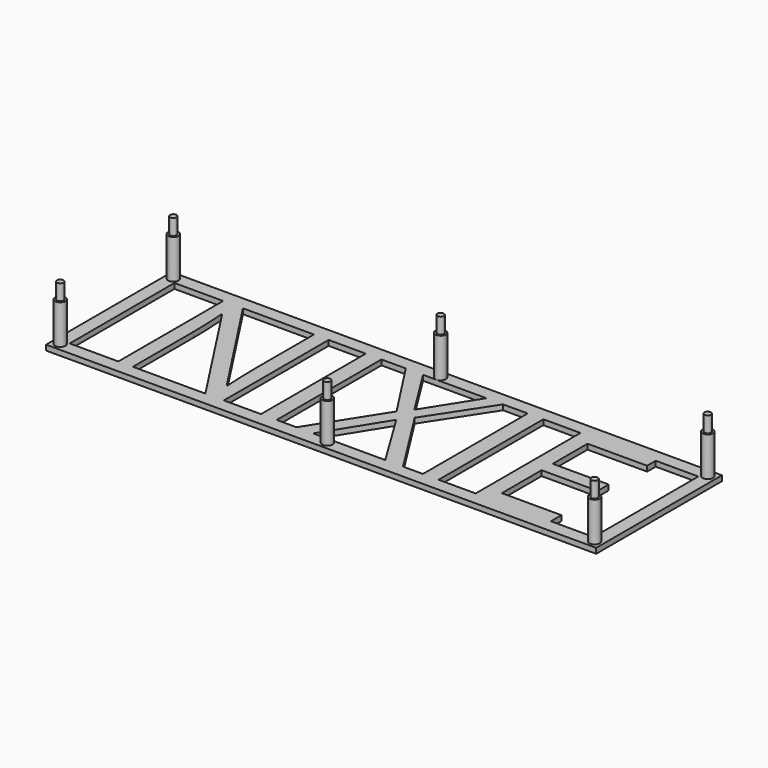
from build123d import *

# Parameters (mm, degrees)
F0_W          = 210
F0_H          = 60
F0_W_2        = 200
F0_H_2        = 50
F1_DEPTH      = 2
F2_R          = 2
F3_DEPTH      = 15
F4_R          = 1.25
F5_DEPTH      = 6
F6_R          = 1.25
F7_DEPTH      = 6
F8_R          = 1.25
F9_DEPTH      = 6
F10_R         = 1.25
F11_DEPTH     = 6
F12_TEXT_SIZE = 72.2222222222
F13_DEPTH     = 2
F14_R         = 1.25
F15_DEPTH     = 6
F16_R         = 1.25
F17_DEPTH     = 6


# Not quite as in the source:
# - a feature names something its author has since deleted; it is built from what else it names
# - Text() gives the source's letters only with a copy of the font that has no kerning and outlines rounded to 1/6400 em; it was checked with that copy


with BuildPart() as f1:
    # F0 (on Top) → F1 (new body)
    with BuildSketch(Plane.XY):
        with Locations((-105, 30)):
            Rectangle(F0_W, F0_H)
        with Locations((-105, 30)):
            Rectangle(F0_W_2, F0_H_2, mode=Mode.SUBTRACT)
    extrude(amount=F1_DEPTH)

    # F2 (on face) → F3 (join)
    with BuildSketch(Plane.XY.offset(2)):
        with Locations((-207, 3)):
            Circle(F2_R)
        with Locations((-207, 57)):
            Circle(F2_R)
        with Locations((-3, 57)):
            Circle(F2_R)
        with Locations((-3, 3)):
            Circle(F2_R)
        with Locations((-105, 3)):
            Circle(F2_R)
        with Locations((-105, 57)):
            Circle(F2_R)
    extrude(amount=F3_DEPTH)

    # F4 (on face) → F5 (join)
    with BuildSketch(Plane.XY.offset(17)):
        with Locations((-207, 3)):
            Circle(F4_R)
    extrude(amount=F5_DEPTH)

    # F6 (on face) → F7 (join)
    with BuildSketch(Plane.XY.offset(17)):
        with Locations((-3, 3)):
            Circle(F6_R)
    extrude(amount=F7_DEPTH)

    # F8 (on face) → F9 (join)
    with BuildSketch(Plane.XY.offset(17)):
        with Locations((-3, 57)):
            Circle(F8_R)
    extrude(amount=F9_DEPTH)

    # F10 (on face) → F11 (join)
    with BuildSketch(Plane.XY.offset(17)):
        with Locations((-207, 57)):
            Circle(F10_R)
    extrude(amount=F11_DEPTH)

    # F12 (on Top) → F13 (join)
    with BuildSketch(Plane.XY):
        with Locations((-193.5, 4.6613515959)):
            Text('NIXIE', F12_TEXT_SIZE, font='Open Sans', text_align=(TextAlign.LEFT, TextAlign.BOTTOM))
    extrude(amount=F13_DEPTH)

    # F14 (on face) → F15 (join)
    with BuildSketch(Plane.XY.offset(17)):
        with Locations((-105, 3)):
            Circle(F14_R)
    extrude(amount=F15_DEPTH)

    # F16 (on face) → F17 (join)
    with BuildSketch(Plane.XY.offset(17)):
        with Locations((-105, 57)):
            Circle(F16_R)
    extrude(amount=F17_DEPTH)


solid = f1.part
